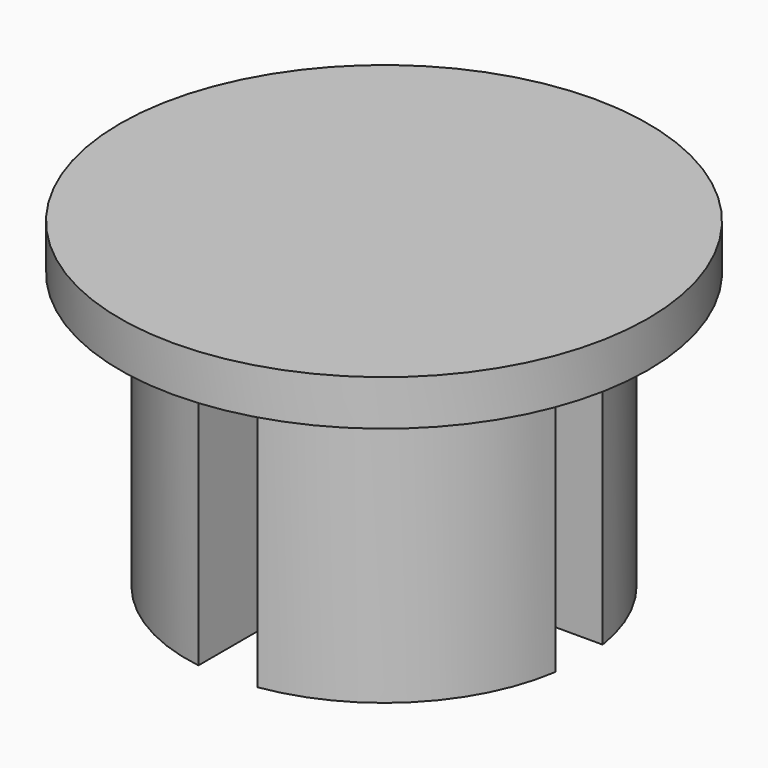
from build123d import *

# Parameters (mm, degrees)
F1_DEPTH = 14
F2_R     = 13.3833019173
F3_DEPTH = 2.3


with BuildPart() as f1:
    # F0 (on Top) → F1 (new body)
    with BuildSketch(Plane.XY):
        with BuildLine():
            Line((1.5, 1.5), (9.8868599666, 1.5))
            ThreePointArc((9.8868599666, 1.5), (7.0710678119, 7.0710678119), (1.5, 9.8868599666))
            Line((1.5, 9.8868599666), (1.5, 1.5))
        make_face()
    extrude(amount=F1_DEPTH)



with BuildPart() as f1b:
    # F0 (on Top) → F1, piece 2 (new body)
    with BuildSketch(Plane.XY):
        with BuildLine():
            ThreePointArc((1.5, -9.8868599666), (7.0710678119, -7.0710678119), (9.8868599666, -1.5))
            Line((9.8868599666, -1.5), (1.5, -1.5))
            Line((1.5, -1.5), (1.5, -9.8868599666))
        make_face()
    extrude(amount=F1_DEPTH)


with BuildPart() as f1c:
    # F0 (on Top) → F1, piece 3 (new body)
    with BuildSketch(Plane.XY):
        with BuildLine():
            Line((-1.5, 1.5), (-1.5, 9.8868599666))
            ThreePointArc((-1.5, 9.8868599666), (-7.0710678119, 7.0710678119), (-9.8868599666, 1.5))
            Line((-9.8868599666, 1.5), (-1.5, 1.5))
        make_face()
    extrude(amount=F1_DEPTH)


with BuildPart() as f1d:
    # F0 (on Top) → F1, piece 4 (new body)
    with BuildSketch(Plane.XY):
        with BuildLine():
            ThreePointArc((-9.8868599666, -1.5), (-7.0710678119, -7.0710678119), (-1.5, -9.8868599666))
            Line((-1.5, -9.8868599666), (-1.5, -1.5))
            Line((-1.5, -1.5), (-9.8868599666, -1.5))
        make_face()
    extrude(amount=F1_DEPTH)


with BuildPart() as f1_1:
    add(f1.part)

    add(f1b.part)  # F3 merges F1b

    add(f1c.part)  # F3 merges F1c

    add(f1d.part)  # F3 merges F1d
    # F2 (on face) → F3 (join)
    with BuildSketch(Plane.XY.offset(14)):
        Circle(F2_R)
        with BuildLine():
            Line((-1.5, 1.5), (-9.8868599666, 1.5))
            ThreePointArc((-9.8868599666, 1.5), (-7.0710678119, 7.0710678119), (-1.5, 9.8868599666))
            Line((-1.5, 9.8868599666), (-1.5, 1.5))
        make_face(mode=Mode.SUBTRACT)
        with BuildLine():
            ThreePointArc((-1.5, 9.8868599666), (-7.0710678119, 7.0710678119), (-9.8868599666, 1.5))
            Line((-9.8868599666, 1.5), (-1.5, 1.5))
            Line((-1.5, 1.5), (-1.5, 9.8868599666))
        make_face()
    extrude(amount=F3_DEPTH)


solid = f1_1.part
